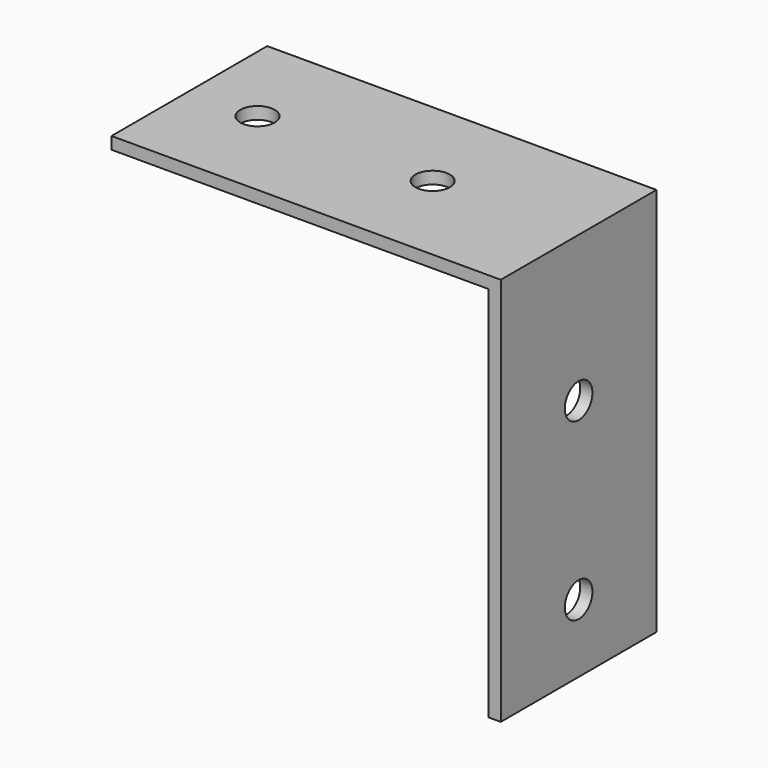
from build123d import *

# Parameters (mm, degrees)
F0_W     = 50.8
F0_H     = 25.4
F1_DEPTH = 1.5875
F2_D     = 4.4958
F3_W     = 25.4
F3_H     = 50.8
F4_DEPTH = 1.5875
F5_D     = 4.4958


# Not quite as in the source:
# - a length typed as a fraction of an inch, garbled in the dataset ("3 / 203.2 mm" for 3/8 in), is restored


with BuildPart() as f1:
    # F0 (on Top) → F1 (new body)
    with BuildSketch(Plane.XY):
        with Locations((6.3499998267, -2.3812473148)):
            Rectangle(F0_W, F0_H)
    extrude(amount=F1_DEPTH)

    # F2 (through all)
    with Locations(Plane(origin=(0, 0, 0), x_dir=(1, 0, 0), z_dir=(0, 0, -1))):
        with Locations((-10.1600001733, 2.3812473148), (12.6999998267, 2.3812473148)):
            Hole(F2_D / 2)

    # F3 (on face) → F4 (join)
    with BuildSketch(Plane.YZ.offset(31.7499998267)):
        with Locations((-2.3812473148, -23.8125)):
            Rectangle(F3_W, F3_H)
    extrude(amount=-F4_DEPTH)

    # F5 (through all)
    with Locations(Plane.YZ.offset(31.7499998267)):
        with Locations((-2.3812473148, -17.4625), (-2.3812473148, -40.3225)):
            Hole(F5_D / 2)


solid = f1.part
